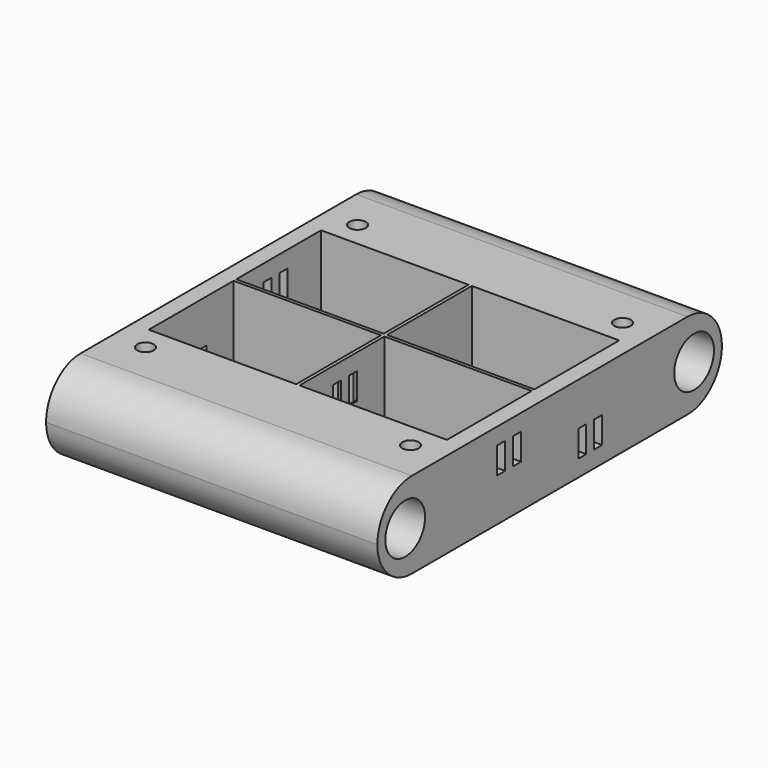
from build123d import *

# Parameters (mm, degrees)
F0_R          = 2.5
F0_W          = 44.5
F0_H          = 1
F0_W_2        = 1
F0_H_2        = 32
F1_DEPTH      = 13
F2_R          = 7.5
F3_DEPTH      = 50
F4_R          = 12.99999
F2_W          = 3
F2_H          = 8
F5_DEPTH      = 50
F6_DEPTH      = 50
F6_DEPTH_BACK = 25


# Not quite as in the source:
# - a fillet or chamfer is up to 0.001 mm smaller than in the source, because OpenCascade refuses the exact size
# - a feature names something its author has since deleted; it is built from what else it names


with BuildPart() as f1:
    # F0 (on Top) → F1 (new body, symmetric)
    with BuildSketch(Plane.XY):
        Polygon((50, 45), (50, 65), (-40, 65), (-50, 65), (-50, -45), (-40, -45), (50, -45), (50, -34.6913893335), (50, 40), align=None)
        with Locations((-40, -40)):
            Circle(F0_R, mode=Mode.SUBTRACT)
        with Locations((40, -40)):
            Circle(F0_R, mode=Mode.SUBTRACT)
        with Locations((-40, 40)):
            Circle(F0_R, mode=Mode.SUBTRACT)
        Polygon((0.5, 32.5), (45, 32.5), (45, 0.5), (45, -0.5), (45, -32.5), (0.5, -32.5), (-0.5, -32.5), (-45, -32.5), (-45, -0.5), (-45, 0.5), (-45, 32.5), (-0.5, 32.5), align=None, mode=Mode.SUBTRACT)
        with Locations((40, 40)):
            Circle(F0_R, mode=Mode.SUBTRACT)
        Polygon((-40, -45), (-50, -45), (-50, -65), (50, -65), (50, -45), align=None)
        with Locations((22.75, 0)):
            Rectangle(F0_W, F0_H)
        with Locations((-22.75, 0)):
            Rectangle(F0_W, F0_H)
        Rectangle(F0_W_2, F0_H)
        with Locations((0, -16.5)):
            Rectangle(F0_W_2, F0_H_2)
        with Locations((0, 16.5)):
            Rectangle(F0_W_2, F0_H_2)
    extrude(amount=F1_DEPTH, both=True)

    # F2 (on Right) → F3 (cut, symmetric)
    with BuildSketch(Plane.YZ):
        with Locations((54.5, 0)):
            Circle(F2_R)
        with Locations((-54.5, 0)):
            Circle(F2_R)
    extrude(amount=F3_DEPTH, both=True, mode=Mode.SUBTRACT)

    # F4 (radius 13 in the source; OpenCascade refuses exactly that, so slightly less here)
    f4_edges = [f1.edges().sort_by_distance(p)[0] for p in [
        (0, 65, 13),
        (0, 65, -13),
        (0, -65, 13),
        (0, -65, -13),
    ]]
    fillet(f4_edges, radius=F4_R)

    # F2 (on Right) → F5 (cut)
    with BuildSketch(Plane.YZ):
        with Locations((-18.3, -4)):
            Rectangle(F2_W, F2_H)
        with Locations((-12.3, -4)):
            Rectangle(F2_W, F2_H)
        with Locations((12.3, 4)):
            Rectangle(F2_W, F2_H)
        with Locations((18.3, 4)):
            Rectangle(F2_W, F2_H)
    extrude(amount=-F5_DEPTH, mode=Mode.SUBTRACT)

    # F2 (on Right) → F6 (cut, two sides)
    with BuildSketch(Plane.YZ) as f6_sk:
        with Locations((12.3, -4)):
            Rectangle(F2_W, F2_H)
        with Locations((18.3, -4)):
            Rectangle(F2_W, F2_H)
        with Locations((-12.3, 4)):
            Rectangle(F2_W, F2_H)
        with Locations((-18.3, 4)):
            Rectangle(F2_W, F2_H)
    extrude(amount=F6_DEPTH, mode=Mode.SUBTRACT)
    extrude(f6_sk.sketch, amount=-F6_DEPTH_BACK, mode=Mode.SUBTRACT)


solid = f1.part
